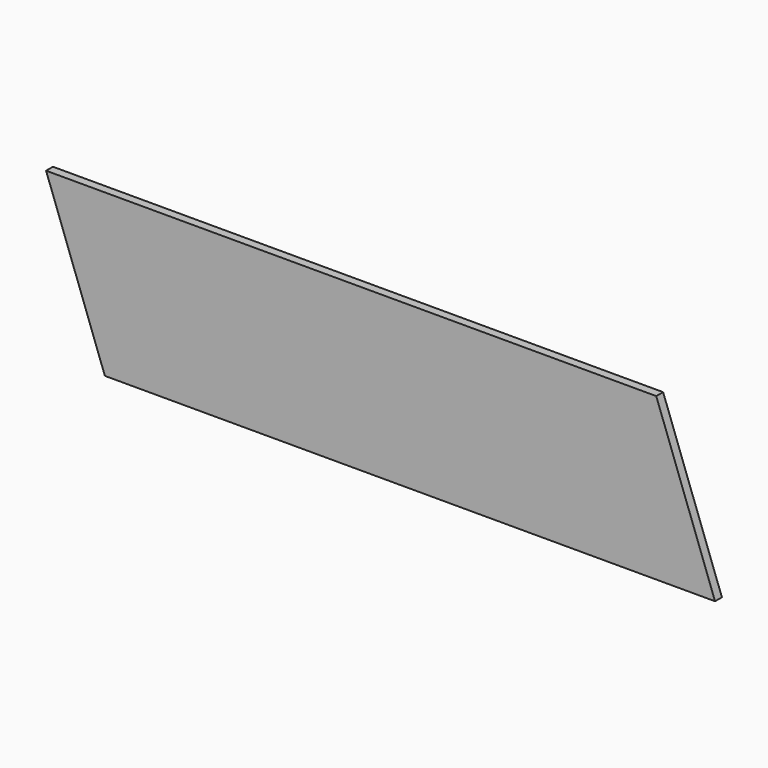
from build123d import *

# Parameters (mm, degrees)
F1_DEPTH = 10


# Not quite as in the source:
# - a feature names something its author has since deleted; it is built from what else it names


with BuildPart() as f1:
    # F0 (on Front) → F1 (new body)
    with BuildSketch(Plane.XZ):
        Polygon((-338.8895529919, -224.8469729066), (-270.4855243268, -412.7854970638), (439.5144756732, -412.7854970638), (371.1104470081, -224.8469729066), align=None)
    extrude(amount=F1_DEPTH)


solid = f1.part
